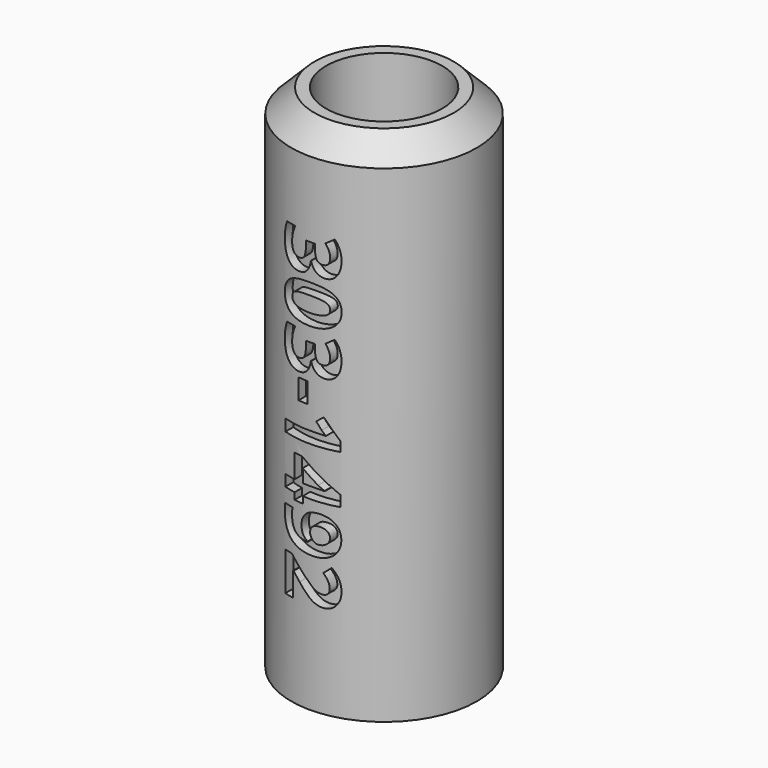
from build123d import *

# Parameters (mm, degrees)
F1_R         = 10
F1_R_2       = 6.25
F2_DEPTH     = 27.5
F3_SIZE      = 2.5
F4_TEXT_SIZE = 8.3333333333
F5_DEPTH     = 25
F6_R         = 9
F6_R_2       = 6.25
F7_DEPTH     = 22.5


# Not quite as in the source:
# - Text() gives the source's letters only with a copy of the font that has no kerning and outlines rounded to 1/6400 em; it was checked with that copy


with BuildPart() as f2:
    # F1 (on Top) → F2 (new body, symmetric)
    with BuildSketch(Plane.XY):
        Circle(F1_R)
        Circle(F1_R_2, mode=Mode.SUBTRACT)
    extrude(amount=F2_DEPTH, both=True)

    # F3
    f3_edges = [f2.edges().sort_by_distance(p)[0] for p in [
        (-10, 0, 27.5),
    ]]
    chamfer(f3_edges, length=F3_SIZE)

    # F4 (on Front) → F5 (cut)
    with BuildSketch(Plane.XZ):
        with Locations(Location((-3, 18.1263020833), (0, 0, -90))):
            Text('303-1492', F4_TEXT_SIZE, font='Open Sans', font_style=FontStyle.BOLD, text_align=(TextAlign.LEFT, TextAlign.BOTTOM))
    extrude(amount=F5_DEPTH, mode=Mode.SUBTRACT)

    # F6 (on Top) → F7 (join, symmetric)
    with BuildSketch(Plane.XY):
        Circle(F6_R)
        Circle(F6_R_2, mode=Mode.SUBTRACT)
    extrude(amount=F7_DEPTH, both=True)


solid = f2.part
